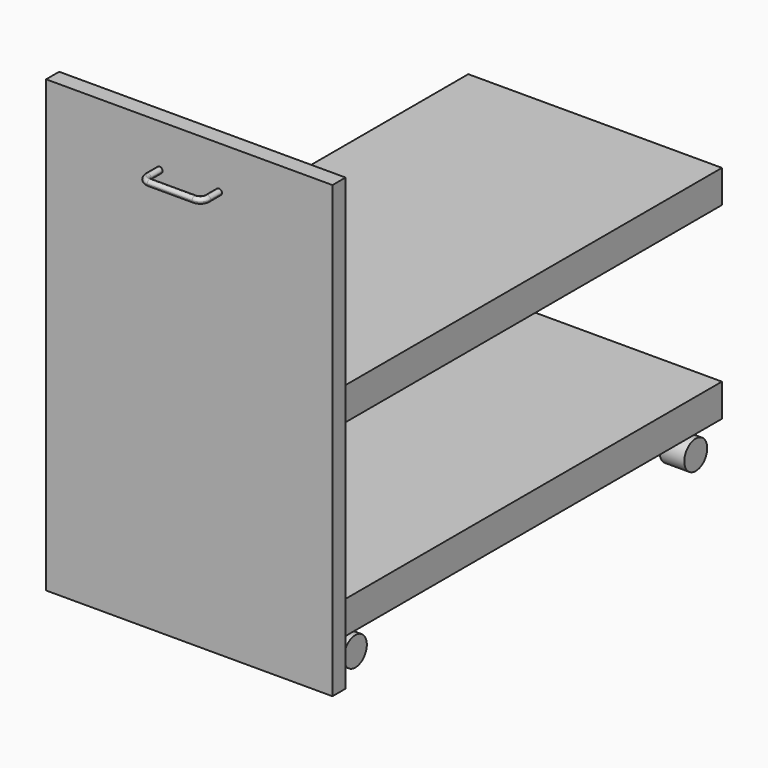
from build123d import *

# Parameters (mm, degrees)
F0_W          = 444.5
F0_H          = 698.5
F1_DEPTH      = 25.4
F2_W          = 393.7
F2_H          = 50.8
F3_DEPTH      = 762
F4_R          = 22.225
F5_DEPTH      = 38.1
F8_DEPTH      = 9.525
F10_T1_DEPTH  = 34.925
F10_T3_DEPTH  = 69.85
F10_T6_ANGLE  = 90
F10_T8_ANGLE  = 90
F10_T10_ANGLE = 90
F10_T12_ANGLE = 90
F10_T14_ANGLE = 90
F10_T16_ANGLE = 90
F10_T18_ANGLE = 90
F10_T20_ANGLE = 90


# Not quite as in the source:
# - a fillet or chamfer that OpenCascade refuses, or shapes differently, is made with other operations: its cross-section is extruded or revolved along the edge and cut away or added


with BuildPart() as f1:
    # F0 (on Front) → F1 (new body)
    with BuildSketch(Plane.XZ):
        with Locations((0, 349.25)):
            Rectangle(F0_W, F0_H)
    extrude(amount=F1_DEPTH)

    # F2 (on face) → F3 (join)
    with BuildSketch(Plane(origin=(0, 0, 0), x_dir=(-1, 0, 0), z_dir=(0, 1, 0))):
        with Locations((0, 368.3)):
            Rectangle(F2_W, F2_H)
        with Locations((0, 76.2)):
            Rectangle(F2_W, F2_H)
    extrude(amount=F3_DEPTH)


with BuildPart() as f5:
    # F4 (on face) → F5 (new body)
    with BuildSketch(Plane.YZ.offset(196.85)):
        with Locations((50.8, 22.225)):
            Circle(F4_R)
    extrude(amount=-F5_DEPTH)


with BuildPart() as f5b:
    # F4 (on face) → F5, piece 2 (new body)
    with BuildSketch(Plane.YZ.offset(196.85)):
        with Locations((711.2, 22.225)):
            Circle(F4_R)
    extrude(amount=-F5_DEPTH)


with BuildPart() as f6_1:
    # F6: instance of F5
    add(f5.part.mirror(Plane.YZ))


with BuildPart() as f6_2:
    # F6: instance of F5b
    add(f5b.part.mirror(Plane.YZ))


with BuildPart() as f8:
    # F7 (on Top) → F8 (new body)
    with BuildSketch(Plane.XY):
        with BuildLine():
            Line((-41.275, -25.4), (-50.8, -25.4))
            Line((-50.8, -25.4), (-50.8, -47.625))
            ThreePointArc((-50.8, -47.625), (-46.1503201513, -58.8503201513), (-34.925, -63.5))
            Line((-34.925, -63.5), (34.925, -63.5))
            ThreePointArc((34.925, -63.5), (46.1503201513, -58.8503201513), (50.8, -47.625))
            Line((50.8, -47.625), (50.8, -25.4))
            Line((50.8, -25.4), (41.275, -25.4))
            Line((41.275, -25.4), (41.275, -47.625))
            ThreePointArc((41.275, -47.625), (39.4151280605, -52.1151280605), (34.925, -53.975))
            Line((34.925, -53.975), (-34.925, -53.975))
            ThreePointArc((-34.925, -53.975), (-39.4151280605, -52.1151280605), (-41.275, -47.625))
            Line((-41.275, -47.625), (-41.275, -25.4))
        make_face()
    extrude(amount=F8_DEPTH)


with BuildPart() as f8_1:
    # F9: moved
    add(f8.part.moved(Location((0, 0, 627.1708))))

    # F10: fillet of radius 5.08 on 4 edges, made by hand

    # F10_s2 → F10_t1 (cut)
    with BuildSketch(Plane.XZ.offset(12.7)):
        with BuildLine():
            ThreePointArc((-41.275, 631.6158), (-42.7628975516, 635.2079024484), (-46.355, 636.6958))
            Line((-46.355, 636.6958), (-41.275, 636.6958))
            Line((-41.275, 636.6958), (-41.275, 631.6158))
        make_face()
        with BuildLine():
            ThreePointArc((-50.8, 631.6158), (-49.3121024484, 635.2079024484), (-45.72, 636.6958))
            Line((-45.72, 636.6958), (-50.8, 636.6958))
            Line((-50.8, 636.6958), (-50.8, 631.6158))
        make_face()
        with BuildLine():
            ThreePointArc((-41.275, 632.2508), (-42.7628975516, 628.6586975516), (-46.355, 627.1708))
            Line((-46.355, 627.1708), (-41.275, 627.1708))
            Line((-41.275, 627.1708), (-41.275, 632.2508))
        make_face()
        with BuildLine():
            ThreePointArc((50.8, 632.2508), (49.3121024484, 628.6586975516), (45.72, 627.1708))
            Line((45.72, 627.1708), (50.8, 627.1708))
            Line((50.8, 627.1708), (50.8, 632.2508))
        make_face()
        with BuildLine():
            ThreePointArc((-50.8, 632.2508), (-49.3121024484, 628.6586975516), (-45.72, 627.1708))
            Line((-45.72, 627.1708), (-50.8, 627.1708))
            Line((-50.8, 627.1708), (-50.8, 632.2508))
        make_face()
        with BuildLine():
            ThreePointArc((41.275, 632.2508), (42.7628975516, 628.6586975516), (46.355, 627.1708))
            Line((46.355, 627.1708), (41.275, 627.1708))
            Line((41.275, 627.1708), (41.275, 632.2508))
        make_face()
        with BuildLine():
            ThreePointArc((50.8, 631.6158), (49.3121024484, 635.2079024484), (45.72, 636.6958))
            Line((45.72, 636.6958), (50.8, 636.6958))
            Line((50.8, 636.6958), (50.8, 631.6158))
        make_face()
        with BuildLine():
            ThreePointArc((41.275, 631.6158), (42.7628975516, 635.2079024484), (46.355, 636.6958))
            Line((46.355, 636.6958), (41.275, 636.6958))
            Line((41.275, 636.6958), (41.275, 631.6158))
        make_face()
    extrude(amount=F10_T1_DEPTH, mode=Mode.SUBTRACT)

    # F10_s4 → F10_t3 (cut)
    with BuildSketch(Plane.YZ.offset(-34.925)):
        with BuildLine():
            ThreePointArc((-63.5, 632.2508), (-62.0121024484, 628.6586975516), (-58.42, 627.1708))
            Line((-58.42, 627.1708), (-63.5, 627.1708))
            Line((-63.5, 627.1708), (-63.5, 632.2508))
        make_face()
        with BuildLine():
            ThreePointArc((-53.975, 632.2508), (-55.4628975516, 628.6586975516), (-59.055, 627.1708))
            Line((-59.055, 627.1708), (-53.975, 627.1708))
            Line((-53.975, 627.1708), (-53.975, 632.2508))
        make_face()
        with BuildLine():
            ThreePointArc((-63.5, 631.6158), (-62.0121024484, 635.2079024484), (-58.42, 636.6958))
            Line((-58.42, 636.6958), (-63.5, 636.6958))
            Line((-63.5, 636.6958), (-63.5, 631.6158))
        make_face()
        with BuildLine():
            ThreePointArc((-53.975, 631.6158), (-55.4628975516, 635.2079024484), (-59.055, 636.6958))
            Line((-59.055, 636.6958), (-53.975, 636.6958))
            Line((-53.975, 636.6958), (-53.975, 631.6158))
        make_face()
    extrude(amount=F10_T3_DEPTH, mode=Mode.SUBTRACT)

    # F10_s5 → F10_t6 (revolve, cut)
    with BuildSketch(Plane.XZ.offset(47.625)):
        with BuildLine():
            ThreePointArc((-50.8, 632.2508), (-49.3121024484, 628.6586975516), (-45.72, 627.1708))
            Line((-45.72, 627.1708), (-50.8, 627.1708))
            Line((-50.8, 627.1708), (-50.8, 632.2508))
        make_face()
    revolve(axis=Axis((-34.925, -47.625, 627.1708), (0, 0, 1)), revolution_arc=F10_T6_ANGLE, mode=Mode.SUBTRACT)

    # F10_s7 → F10_t8 (revolve, cut)
    with BuildSketch(Plane.YZ.offset(34.925)):
        with BuildLine():
            ThreePointArc((-63.5, 632.2508), (-62.0121024484, 628.6586975516), (-58.42, 627.1708))
            Line((-58.42, 627.1708), (-63.5, 627.1708))
            Line((-63.5, 627.1708), (-63.5, 632.2508))
        make_face()
    revolve(axis=Axis((34.925, -47.625, 627.1708), (0, 0, 1)), revolution_arc=F10_T8_ANGLE, mode=Mode.SUBTRACT)

    # F10_s9 → F10_t10 (revolve, cut)
    with BuildSketch(Plane.YZ.offset(-34.925)):
        with BuildLine():
            ThreePointArc((-53.975, 632.2508), (-55.4628975516, 628.6586975516), (-59.055, 627.1708))
            Line((-59.055, 627.1708), (-53.975, 627.1708))
            Line((-53.975, 627.1708), (-53.975, 632.2508))
        make_face()
    revolve(axis=Axis((-34.925, -47.625, 627.1708), (0, 0, -1)), revolution_arc=F10_T10_ANGLE, mode=Mode.SUBTRACT)

    # F10_s11 → F10_t12 (revolve, cut)
    with BuildSketch(Plane.XZ.offset(47.625)):
        with BuildLine():
            ThreePointArc((41.275, 632.2508), (42.7628975516, 628.6586975516), (46.355, 627.1708))
            Line((46.355, 627.1708), (41.275, 627.1708))
            Line((41.275, 627.1708), (41.275, 632.2508))
        make_face()
    revolve(axis=Axis((34.925, -47.625, 627.1708), (0, 0, -1)), revolution_arc=F10_T12_ANGLE, mode=Mode.SUBTRACT)

    # F10_s13 → F10_t14 (revolve, cut)
    with BuildSketch(Plane.XZ.offset(47.625)):
        with BuildLine():
            ThreePointArc((-50.8, 631.6158), (-49.3121024484, 635.2079024484), (-45.72, 636.6958))
            Line((-45.72, 636.6958), (-50.8, 636.6958))
            Line((-50.8, 636.6958), (-50.8, 631.6158))
        make_face()
    revolve(axis=Axis((-34.925, -47.625, 636.6958), (0, 0, 1)), revolution_arc=F10_T14_ANGLE, mode=Mode.SUBTRACT)

    # F10_s15 → F10_t16 (revolve, cut)
    with BuildSketch(Plane.YZ.offset(34.925)):
        with BuildLine():
            ThreePointArc((-63.5, 631.6158), (-62.0121024484, 635.2079024484), (-58.42, 636.6958))
            Line((-58.42, 636.6958), (-63.5, 636.6958))
            Line((-63.5, 636.6958), (-63.5, 631.6158))
        make_face()
    revolve(axis=Axis((34.925, -47.625, 636.6958), (0, 0, 1)), revolution_arc=F10_T16_ANGLE, mode=Mode.SUBTRACT)

    # F10_s17 → F10_t18 (revolve, cut)
    with BuildSketch(Plane.YZ.offset(-34.925)):
        with BuildLine():
            ThreePointArc((-53.975, 631.6158), (-55.4628975516, 635.2079024484), (-59.055, 636.6958))
            Line((-59.055, 636.6958), (-53.975, 636.6958))
            Line((-53.975, 636.6958), (-53.975, 631.6158))
        make_face()
    revolve(axis=Axis((-34.925, -47.625, 636.6958), (0, 0, -1)), revolution_arc=F10_T18_ANGLE, mode=Mode.SUBTRACT)

    # F10_s19 → F10_t20 (revolve, cut)
    with BuildSketch(Plane.XZ.offset(47.625)):
        with BuildLine():
            ThreePointArc((41.275, 631.6158), (42.7628975516, 635.2079024484), (46.355, 636.6958))
            Line((46.355, 636.6958), (41.275, 636.6958))
            Line((41.275, 636.6958), (41.275, 631.6158))
        make_face()
    revolve(axis=Axis((34.925, -47.625, 636.6958), (0, 0, -1)), revolution_arc=F10_T20_ANGLE, mode=Mode.SUBTRACT)


solid = Compound([f1.part, f5.part, f5b.part, f6_1.part, f6_2.part, f8_1.part])
